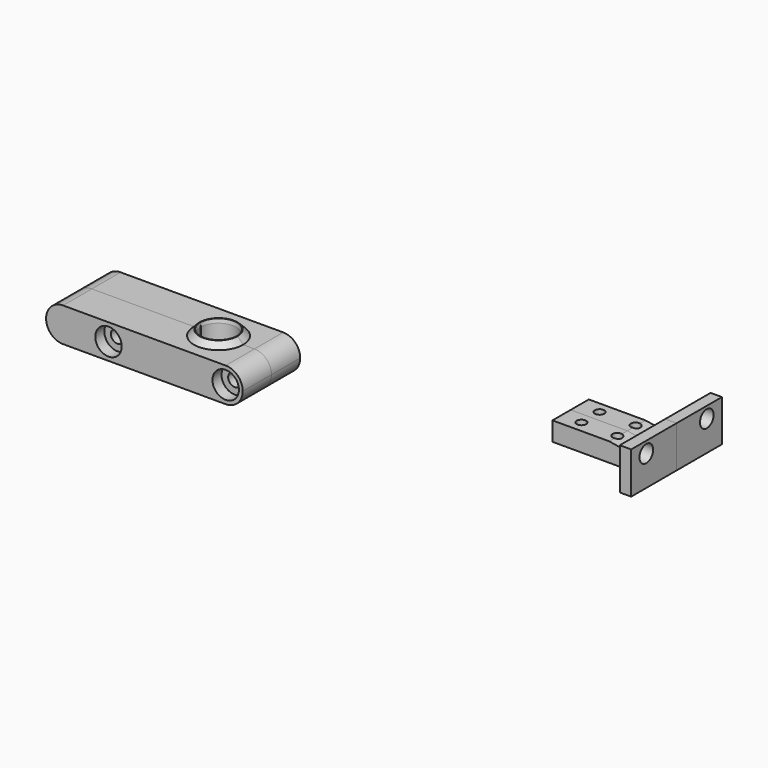
from build123d import *

# Parameters (mm, degrees)
F0_W           = 52
F0_H           = 9
F1_DEPTH       = 9.5
F3_DEPTH       = 4.5
F4_DEPTH       = 1.5
F5_SIZE        = 1.49999
F6_W           = 3
F6_H           = 2.5
F7_ANGLE       = 180
F10_SIZE2      = 0.74999
F10_SIZE       = 2.49999
F11_R          = 1.75
F12_DEPTH      = 42.06082
F13_R          = 4.49999
F15_R          = 3.5
F15_R_2        = 1.75
F16_DEPTH      = 3
F17_W          = 20
F17_H          = 6
F17_R          = 1.25
F18_DEPTH      = 5
F20_DEPTH      = 15
F21_T4_DEPTH   = 51.5816860873
F22_R          = 2.25
F23_DEPTH      = 25
F25_DEPTH      = 25
F27_T1_DEPTH   = 6.2546093825
F27_2_T1_DEPTH = 6.2546093825
F28_SIZE2      = 0.2
F28_SIZE       = 1
F29_SIZE2      = 1
F29_SIZE       = 0.2


# Not quite as in the source:
# - a fillet or chamfer that OpenCascade refuses, or shapes differently, is made with other operations: its cross-section is extruded or revolved along the edge and cut away or added
# - a fillet or chamfer is up to 0.001 mm smaller than in the source, because OpenCascade refuses the exact size


with BuildPart() as f1:
    # F0 (on Front) → F1 (new body)
    with BuildSketch(Plane.XZ):
        with Locations((3.196533835, 28.8128983229)):
            Rectangle(F0_W, F0_H)
    extrude(amount=F1_DEPTH)

    # F2 (on face) → F3 (cut)
    with BuildSketch(Plane.XY.offset(33.3128983229)):
        with BuildLine():
            Line((10.546533835, -9.5), (19.846533835, -9.5))
            ThreePointArc((19.846533835, -9.5), (15.196533835, -4.85), (10.546533835, -9.5))
        make_face()
    extrude(amount=-F3_DEPTH, mode=Mode.SUBTRACT)

    # F2 (on face) → F4 (join)
    with BuildSketch(Plane.XY.offset(33.3128983229)):
        with BuildLine():
            ThreePointArc((10.546533835, -9.5), (15.196533835, -4.85), (19.846533835, -9.5))
            Line((19.846533835, -9.5), (21.696533835, -9.5))
            ThreePointArc((21.696533835, -9.5), (15.196533835, -3), (8.696533835, -9.5))
            Line((8.696533835, -9.5), (10.546533835, -9.5))
        make_face()
    extrude(amount=F4_DEPTH)

    # F5 (size 1.5 in the source; OpenCascade refuses exactly that, so slightly less here)
    f5_edges = [f1.edges().sort_by_distance(p)[0] for p in [
        (15.196534, -3, 34.812898),
    ]]
    chamfer(f5_edges, length=F5_SIZE)

    # F6 (on face) → F7 (revolve)
    with BuildSketch(Plane.XZ.offset(9.5)):
        with Locations((16.696533835, 23.0628983229)):
            Rectangle(F6_W, F6_H)
        Polygon((16.196533835, 28.8128983229), (15.196533835, 28.8128983229), (15.196533835, 24.3128983229), (18.196533835, 24.3128983229), align=None)
    revolve(axis=Axis((15.196533835, -9.5, 25.3128983229), (0, 0, 1)), revolution_arc=F7_ANGLE)

    # F8 (on face) → F9 (revolve, cut)
    with BuildSketch(Plane.XZ.offset(9.5)):
        Polygon((16.196533835, 28.8128983229), (15.196533835, 28.8128983229), (15.196533835, 21.8128983229), (17.196533835, 21.8128983229), align=None)
    revolve(axis=Axis((15.196533835, -9.5, 25.3128983229), (0, 0, -1)), mode=Mode.SUBTRACT)

    # F10 (size 2.5 and 0.75 in the source; OpenCascade refuses exactly that, so slightly less here)
    f10_edges = [f1.edges().sort_by_distance(p)[0] for p in [
        (15.196534, -6.5, 21.812898),
    ]]
    f10_side = f1.faces().sort_by_distance((15.196534, -6.5, 23.062898))[0]
    chamfer(f10_edges, length=F10_SIZE, length2=F10_SIZE2, reference=f10_side)

    # F11 (on Front) → F12 (cut)
    with BuildSketch(Plane.XZ):
        with Locations((24.696533835, 28.8128983229)):
            Circle(F11_R)
        with Locations((-6.303466165, 28.8128983229)):
            Circle(F11_R)
    extrude(amount=F12_DEPTH, mode=Mode.SUBTRACT)

    # F13 (radius 4.5 in the source; OpenCascade refuses exactly that, so slightly less here)
    f13_edges = [f1.edges().sort_by_distance(p)[0] for p in [
        (29.196534, -4.75, 33.312898),
        (29.196534, -4.75, 24.312898),
        (-22.803466, -4.75, 33.312898),
        (-22.803466, -4.75, 24.312898),
    ]]
    fillet(f13_edges, radius=F13_R)


with BuildPart() as f14_1:
    # F14: instance of F1
    add(f1.part.mirror(Plane(origin=(-4.5395011787, -9.5, 28.6957157719), x_dir=(1, 0, 0), z_dir=(0, -1, 0))))

    # F15 (on face) → F16 (cut)
    with BuildSketch(Plane.XZ.offset(19)):
        with Locations((-6.303466165, 28.8128983229)):
            Circle(F15_R)
        with Locations((-6.303466165, 28.8128983229)):
            Circle(F15_R_2, mode=Mode.SUBTRACT)
        with Locations((24.696533835, 28.8128983229)):
            Circle(F15_R)
        with Locations((24.696533835, 28.8128983229)):
            Circle(F15_R_2, mode=Mode.SUBTRACT)
    extrude(amount=-F16_DEPTH, mode=Mode.SUBTRACT)

    # F27: chamfer of 0.1 on 2 edges, made by hand

    # F27_s2 → F27_t1 (cut)
    with BuildSketch(Plane.XY.offset(28.8128983229)):
        with BuildLine():
            Line((10.5475644201, -9.5978947368), (10.4475865832, -9.5))
            Line((10.4475865832, -9.5), (10.546533835, -9.5))
            ThreePointArc((10.546533835, -9.5), (10.5468065962, -9.5503647222), (10.5475644201, -9.5978947368))
        make_face()
        with BuildLine():
            Line((19.9454810868, -9.5), (19.8455032499, -9.5978947368))
            ThreePointArc((19.8455032499, -9.5978947368), (19.8462610737, -9.5503647222), (19.846533835, -9.5))
            Line((19.846533835, -9.5), (19.9454810868, -9.5))
        make_face()
    extrude(amount=F27_T1_DEPTH, mode=Mode.SUBTRACT)

    # F28
    f28_edges = [f14_1.edges().sort_by_distance(p)[0] for p in [
        (15.196534, -14.15, 34.812898),
    ]]
    f28_side = f14_1.faces().sort_by_distance((15.196534, -14.15, 31.812898))[0]
    chamfer(f28_edges, length=F28_SIZE, length2=F28_SIZE2, reference=f28_side)


with BuildPart() as f18:
    # F17 (on Top) → F18 (new body)
    with BuildSketch(Plane.XY):
        with Locations((68.7268972397, 55.4795021277)):
            Rectangle(F17_W, F17_H)
        with Locations((63.9768972397, 55.4795021277)):
            Circle(F17_R, mode=Mode.SUBTRACT)
        with Locations((73.4768972397, 55.4795021277)):
            Circle(F17_R, mode=Mode.SUBTRACT)
    extrude(amount=F18_DEPTH)

    # F19 (on face) → F20 (join)
    with BuildSketch(Plane.XZ.offset(-52.4795021277)):
        Polygon((83.7268972397, 5), (78.7268972397, 5), (78.7268972397, 0), (86.7268972397, 0), (86.7268972397, 11), (83.7268972397, 11), align=None)
    extrude(amount=-F20_DEPTH)

    # F21: chamfer of 9 x 5 on 1 edges, made by hand


with BuildPart() as f21_tool2:
    # F21_s3 → F21_t4 (new body)
    with BuildSketch(Plane.XY.offset(28.2908430436)):
        Polygon((83.7268972397, 67.4795021277), (78.7268972397, 58.4795021277), (78.7268972397, 67.4795021277), align=None)
    extrude(amount=-F21_T4_DEPTH)

    split(bisect_by=Plane.XZ.offset(-58.4795021277), keep=Keep.BOTTOM)


with BuildPart() as f18_1:
    add(f18.part)

    # F21_t1: cut F21_tool2
    add(f21_tool2.part, mode=Mode.SUBTRACT)

    # F22 (on face) → F23 (cut)
    with BuildSketch(Plane(origin=(83.7268972397, 0, 0), x_dir=(0, -1, 0), z_dir=(-1, 0, 0))):
        with Locations((-62.4795021277, 8)):
            Circle(F22_R)
    extrude(amount=-F23_DEPTH, mode=Mode.SUBTRACT)

    # F24 (on face) → F25 (cut)
    with BuildSketch(Plane.XZ.offset(-52.4795021277)):
        Polygon((83.7268972397, 4), (83.7268972397, 5), (73.7268972397, 5), (79.7268972397, 4), align=None)
    extrude(amount=-F25_DEPTH, mode=Mode.SUBTRACT)


with BuildPart() as f26_1:
    # F26: instance of F18
    add(f18_1.part.mirror(Plane(origin=(73.8792151205, 52.4795021277, 3.059602649), x_dir=(1, 0, 0), z_dir=(0, -1, 0))))


with BuildPart() as f1_1:
    add(f1.part)

    # F27#2: chamfer of 0.1 on 2 edges, made by hand

    # F27_2_s2 → F27_2_t1 (cut)
    with BuildSketch(Plane.XY.offset(28.8128983229)):
        with BuildLine():
            Line((10.5475644201, -9.4021052632), (10.4475865832, -9.5))
            Line((10.4475865832, -9.5), (10.546533835, -9.5))
            ThreePointArc((10.546533835, -9.5), (10.5468065962, -9.4496352778), (10.5475644201, -9.4021052632))
        make_face()
        with BuildLine():
            Line((19.9454810868, -9.5), (19.8455032499, -9.4021052632))
            ThreePointArc((19.8455032499, -9.4021052632), (19.8462610737, -9.4496352778), (19.846533835, -9.5))
            Line((19.846533835, -9.5), (19.9454810868, -9.5))
        make_face()
    extrude(amount=F27_2_T1_DEPTH, mode=Mode.SUBTRACT)

    # F29
    f29_edges = [f1_1.edges().sort_by_distance(p)[0] for p in [
        (15.196534, -4.85, 34.812898),
    ]]
    f29_side = f1_1.faces().sort_by_distance((15.196534, -4.611794, 34.812898))[0]
    chamfer(f29_edges, length=F29_SIZE, length2=F29_SIZE2, reference=f29_side)


solid = Compound([f14_1.part, f18_1.part, f26_1.part, f1_1.part])
